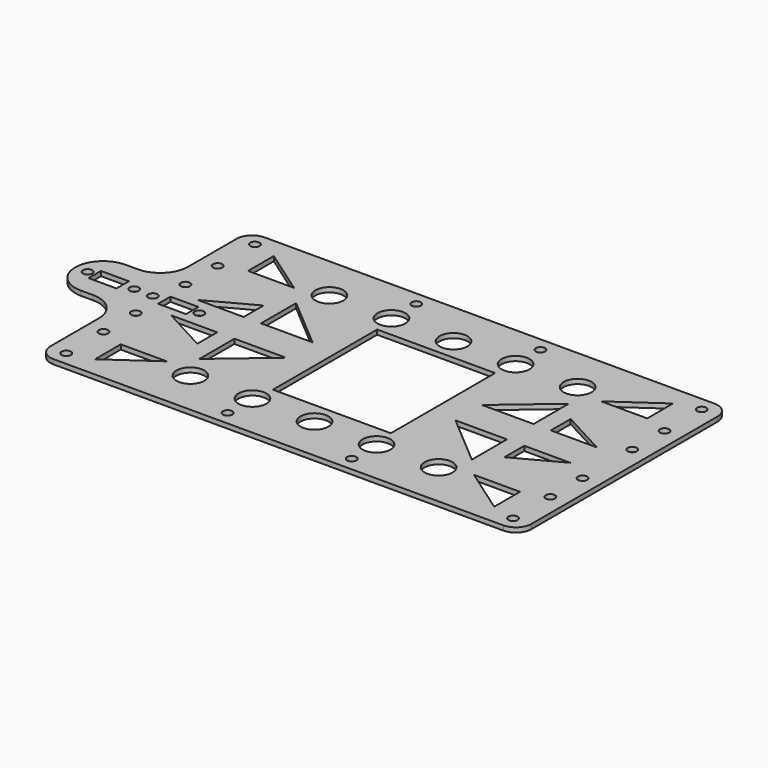
from build123d import *

# Parameters (mm, degrees)
F0_R     = 1.5
F0_R_2   = 4.5
F0_W     = 9
F0_H     = 5
F0_W_2   = 38
F0_H_2   = 42
F0_W_3   = 22
F0_H_3   = 18
F1_DEPTH = 1.5
F2_R     = 5
F3_R     = 8.99999


# Not quite as in the source:
# - a fillet or chamfer is up to 0.001 mm smaller than in the source, because OpenCascade refuses the exact size


with BuildPart() as f1:
    # F0 (on Top) → F1 (new body)
    with BuildSketch(Plane.XY):
        Polygon((-77.5, -42.5), (77.5, -42.5), (77.5, 42.5), (-77.5, 42.5), (-77.5, 9), (-77.5, -9), align=None)
        with Locations((-72, -38)):
            Circle(F0_R, mode=Mode.SUBTRACT)
        Polygon((-49.4840586844, -25.6258432192), (-64.3245950341, -36.0181480646), (-64.3245950341, -25.6258432192), align=None, mode=Mode.SUBTRACT)
        with Locations((-72, -23)):
            Circle(F0_R, mode=Mode.SUBTRACT)
        with Locations((-20, -38)):
            Circle(F0_R, mode=Mode.SUBTRACT)
        with Locations((-40, -28)):
            Circle(F0_R_2, mode=Mode.SUBTRACT)
        with Locations((-20, -28)):
            Circle(F0_R_2, mode=Mode.SUBTRACT)
        with Locations((-72, -10)):
            Circle(F0_R, mode=Mode.SUBTRACT)
        Polygon((-49.4840586844, -13.3469680754), (-64.3245950341, -5.3528225981), (-49.4840586844, -5.3528225981), align=None, mode=Mode.SUBTRACT)
        Polygon((-43.9106635749, -19.5035282522), (-43.9106635749, -5.3528225981), (-27.3078400642, -5.3528225981), align=None, mode=Mode.SUBTRACT)
        with Locations((20, -38)):
            Circle(F0_R, mode=Mode.SUBTRACT)
        with Locations((0, -28)):
            Circle(F0_R_2, mode=Mode.SUBTRACT)
        with Locations((20, -28)):
            Circle(F0_R_2, mode=Mode.SUBTRACT)
        with Locations((72, -38)):
            Circle(F0_R, mode=Mode.SUBTRACT)
        with Locations((40, -28)):
            Circle(F0_R_2, mode=Mode.SUBTRACT)
        Polygon((64.3245950341, -36.0181480646), (49.4840586844, -25.6258432192), (64.3245950341, -25.6258432192), align=None, mode=Mode.SUBTRACT)
        with Locations((72, -23)):
            Circle(F0_R, mode=Mode.SUBTRACT)
        Polygon((43.9106635749, -19.5035282522), (27.3078400642, -5.3528225981), (43.9106635749, -5.3528225981), align=None, mode=Mode.SUBTRACT)
        Polygon((64.3245950341, -5.3528225981), (49.4840586844, -13.3469680754), (49.4840586844, -5.3528225981), align=None, mode=Mode.SUBTRACT)
        with Locations((72, -10)):
            Circle(F0_R, mode=Mode.SUBTRACT)
        with Locations((-74.5, 0)):
            Circle(F0_R, mode=Mode.SUBTRACT)
        with Locations((-66.3017949164, 0)):
            Rectangle(F0_W, F0_H, mode=Mode.SUBTRACT)
        with Locations((-59.5, 0)):
            Circle(F0_R, mode=Mode.SUBTRACT)
        with Locations((-72, 10)):
            Circle(F0_R, mode=Mode.SUBTRACT)
        Polygon((-49.4840586844, 5.3528225981), (-64.3245950341, 5.3528225981), (-49.4840586844, 13.3469680754), align=None, mode=Mode.SUBTRACT)
        Polygon((-43.9106635749, 5.3528225981), (-43.9106635749, 19.5035282522), (-27.3078400642, 5.3528225981), align=None, mode=Mode.SUBTRACT)
        with Locations((-72, 23)):
            Circle(F0_R, mode=Mode.SUBTRACT)
        Polygon((-64.3245950341, 36.0181480646), (-49.4840586844, 25.6258432192), (-64.3245950341, 25.6258432192), align=None, mode=Mode.SUBTRACT)
        with Locations((-72, 38)):
            Circle(F0_R, mode=Mode.SUBTRACT)
        with Locations((-40, 28)):
            Circle(F0_R_2, mode=Mode.SUBTRACT)
        with Locations((-20, 28)):
            Circle(F0_R_2, mode=Mode.SUBTRACT)
        with Locations((-20, 38)):
            Circle(F0_R, mode=Mode.SUBTRACT)
        Rectangle(F0_W_2, F0_H_2, mode=Mode.SUBTRACT)
        Polygon((49.4840586844, 5.3528225981), (49.4840586844, 13.3469680754), (64.3245950341, 5.3528225981), align=None, mode=Mode.SUBTRACT)
        with Locations((72, 10)):
            Circle(F0_R, mode=Mode.SUBTRACT)
        Polygon((43.9106635749, 19.5035282522), (43.9106635749, 5.3528225981), (27.3078400642, 5.3528225981), align=None, mode=Mode.SUBTRACT)
        with Locations((0, 28)):
            Circle(F0_R_2, mode=Mode.SUBTRACT)
        with Locations((20, 28)):
            Circle(F0_R_2, mode=Mode.SUBTRACT)
        with Locations((20, 38)):
            Circle(F0_R, mode=Mode.SUBTRACT)
        with Locations((40, 28)):
            Circle(F0_R_2, mode=Mode.SUBTRACT)
        with Locations((72, 23)):
            Circle(F0_R, mode=Mode.SUBTRACT)
        Polygon((64.3245950341, 25.6258432192), (49.4840586844, 25.6258432192), (64.3245950341, 36.0181480646), align=None, mode=Mode.SUBTRACT)
        with Locations((72, 38)):
            Circle(F0_R, mode=Mode.SUBTRACT)
        with Locations((-88.5, 0)):
            Rectangle(F0_W_3, F0_H_3)
        with Locations((-95.5, 0)):
            Circle(F0_R, mode=Mode.SUBTRACT)
        with Locations((-88.6982050836, 0)):
            Rectangle(F0_W, F0_H, mode=Mode.SUBTRACT)
        with Locations((-80.5, 0)):
            Circle(F0_R, mode=Mode.SUBTRACT)
    extrude(amount=F1_DEPTH)

    # F2
    f2_edges = [f1.edges().sort_by_distance(p)[0] for p in [
        (-77.5, 42.5, 0.75),
        (77.5, 42.5, 0.75),
        (77.5, -42.5, 0.75),
        (-77.5, -42.5, 0.75),
    ]]
    fillet(f2_edges, radius=F2_R)

    # F3 (radius 9 in the source; OpenCascade refuses exactly that, so slightly less here)
    f3_edges = [f1.edges().sort_by_distance(p)[0] for p in [
        (-77.5, -9, 0.75),
        (-77.5, 9, 0.75),
        (-99.5, -9, 0.75),
        (-99.5, 9, 0.75),
    ]]
    fillet(f3_edges, radius=F3_R)


solid = f1.part
